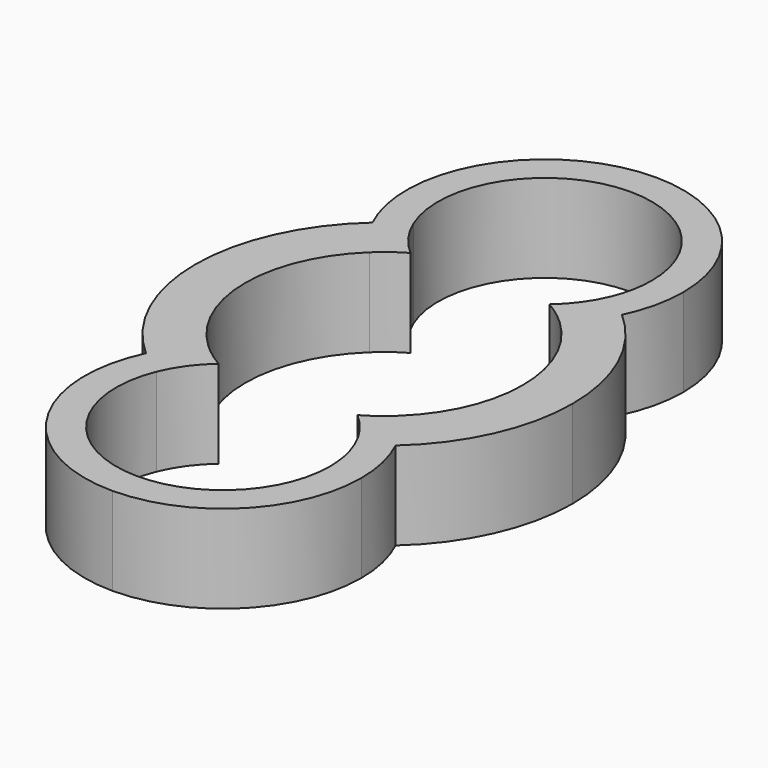
from build123d import *

# Parameters (mm, degrees)
F1_DEPTH = 7


with BuildPart() as f1:
    # F0 (on Top) → F1 (new body)
    with BuildSketch(Plane.XY):
        with BuildLine():
            ThreePointArc((7.5680259261, 8.0172070312), (10.1239347794, 4.3653830969), (11.025, 0))
            ThreePointArc((11.025, 0), (10.1239347794, -4.3653830969), (7.5680259261, -8.0172070312))
            ThreePointArc((7.5680259261, -8.0172070313), (8.8929301367, -9.5257592273), (9.9215674165, -11.25))
            ThreePointArc((9.9215674165, -11.25), (13.6715674165, -6.1715674165), (15, 0))
            ThreePointArc((15, 0), (13.6715674165, 6.1715674165), (9.9215674165, 11.25))
            ThreePointArc((9.9215674165, 11.25), (8.8929301367, 9.5257592273), (7.5680259261, 8.0172070312))
        make_face()
        with BuildLine():
            ThreePointArc((5.5250997211, 9.5406445313), (6.5907283556, 8.8381516587), (7.5680259261, 8.0172070312))
            ThreePointArc((7.5680259261, 8.0172070312), (8.8929301367, 9.5257592273), (9.9215674165, 11.25))
            ThreePointArc((9.9215674165, 11.25), (8.9252455049, 12.0557037405), (7.863796439, 12.7734375))
            ThreePointArc((7.863796439, 12.7734375), (6.8868260245, 11.0178691999), (5.5250997211, 9.5406445312))
        make_face()
        with BuildLine():
            ThreePointArc((9.9215674165, -11.25), (8.8929301367, -9.5257592273), (7.5680259261, -8.0172070313))
            ThreePointArc((7.5680259261, -8.0172070312), (6.5907283556, -8.8381516587), (5.5250997211, -9.5406445313))
            ThreePointArc((5.5250997211, -9.5406445312), (6.8868260245, -11.0178691999), (7.863796439, -12.7734375))
            ThreePointArc((7.863796439, -12.7734375), (8.9252455049, -12.0557037405), (9.9215674165, -11.25))
        make_face()
        with BuildLine():
            ThreePointArc((7.863796439, 12.7734375), (8.9252455049, 12.0557037405), (9.9215674165, 11.25))
            ThreePointArc((9.9215674165, 11.25), (10.7270042785, 13.5645576974), (11, 16))
            ThreePointArc((11, 16), (7.7781745931, 23.7781745931), (0, 27))
            Line((0, 27), (0, 24.5))
            ThreePointArc((0, 24.5), (6.0104076401, 22.0104076401), (8.5, 16))
            ThreePointArc((8.5, 16), (8.3394325266, 14.3556566252), (7.863796439, 12.7734375))
        make_face()
        with BuildLine():
            ThreePointArc((11, -16), (10.7270042785, -13.5645576974), (9.9215674165, -11.25))
            ThreePointArc((9.9215674165, -11.25), (8.9252455049, -12.0557037405), (7.863796439, -12.7734375))
            ThreePointArc((7.863796439, -12.7734375), (8.3394325266, -14.3556566252), (8.5, -16))
            ThreePointArc((8.5, -16), (6.0104076401, -22.0104076401), (0, -24.5))
            Line((0, -24.5), (0, -27))
            ThreePointArc((0, -27), (7.7781745931, -23.7781745931), (11, -16))
        make_face()
        with BuildLine():
            ThreePointArc((-9.9215674165, 11.25), (-8.8929301367, 9.5257592273), (-7.5680259261, 8.0172070313))
            ThreePointArc((-7.5680259261, 8.0172070312), (-6.5907283556, 8.8381516587), (-5.5250997211, 9.5406445313))
            ThreePointArc((-5.5250997211, 9.5406445312), (-6.8868260245, 11.0178691999), (-7.863796439, 12.7734375))
            ThreePointArc((-7.863796439, 12.7734375), (-8.9252455049, 12.0557037405), (-9.9215674165, 11.25))
        make_face()
        with BuildLine():
            ThreePointArc((-7.5680259261, -8.0172070312), (-11.025, 0), (-7.5680259261, 8.0172070312))
            ThreePointArc((-7.5680259261, 8.0172070313), (-8.8929301367, 9.5257592273), (-9.9215674165, 11.25))
            ThreePointArc((-9.9215674165, 11.25), (-15, 0), (-9.9215674165, -11.25))
            ThreePointArc((-9.9215674165, -11.25), (-8.8929301367, -9.5257592273), (-7.5680259261, -8.0172070313))
        make_face()
        with BuildLine():
            ThreePointArc((-5.5250997211, -9.5406445313), (-6.5907283556, -8.8381516587), (-7.5680259261, -8.0172070312))
            ThreePointArc((-7.5680259261, -8.0172070313), (-8.8929301367, -9.5257592273), (-9.9215674165, -11.25))
            ThreePointArc((-9.9215674165, -11.25), (-8.9252455049, -12.0557037405), (-7.863796439, -12.7734375))
            ThreePointArc((-7.863796439, -12.7734375), (-6.8868260245, -11.0178691999), (-5.5250997211, -9.5406445312))
        make_face()
        with BuildLine():
            ThreePointArc((0, 27), (-9.3072552345, 21.8630196998), (-9.9215674165, 11.25))
            ThreePointArc((-9.9215674165, 11.25), (-8.9252455049, 12.0557037405), (-7.863796439, 12.7734375))
            ThreePointArc((-7.863796439, 12.7734375), (-7.0595956417, 20.7341429399), (0, 24.5))
            Line((0, 24.5), (0, 27))
        make_face()
        with BuildLine():
            ThreePointArc((-9.9215674165, -11.25), (-9.3072552345, -21.8630196998), (0, -27))
            Line((0, -27), (0, -24.5))
            ThreePointArc((0, -24.5), (-7.0595956417, -20.7341429399), (-7.863796439, -12.7734375))
            ThreePointArc((-7.863796439, -12.7734375), (-8.9252455049, -12.0557037405), (-9.9215674165, -11.25))
        make_face()
    extrude(amount=F1_DEPTH)


solid = f1.part
